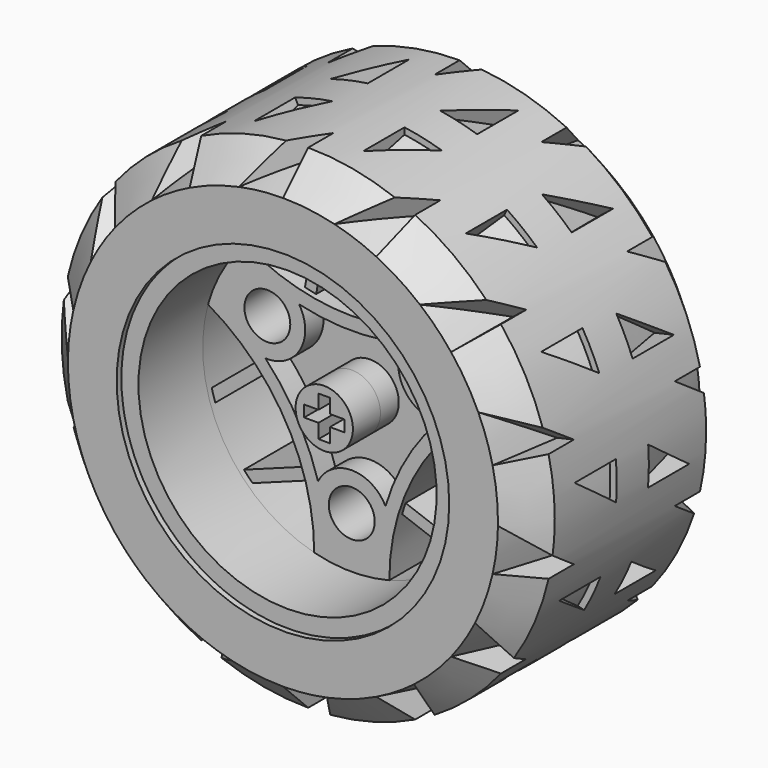
from build123d import *

# Parameters (mm, degrees)
F0_R             = 21.5
F0_R_2           = 14.5
F1_DEPTH         = 11
F1_DEPTH_BACK    = 11
F6_DEPTH         = 3.5
F6_COPIES_COUNT  = 14
F9_COPIES_COUNT  = 2
F11_COPIES_COUNT = 2
F14_R            = 2
F15_DEPTH        = 25
F16_R            = 2.5
F17_DEPTH        = 3
F19_DEPTH        = 17.501
F20_R            = 2.5
F21_DEPTH        = 2
F24_DEPTH        = 6
F24_COPIES_COUNT = 3


# Not quite as in the source:
# - a pattern or mirror of a feature is missing from the dataset's text; its kind, count and spacing are read off the source's solid


with BuildPart() as f1:
    # F0 (on Front) → F1 (new body, two sides)
    with BuildSketch(Plane.XZ) as f1_sk:
        Circle(F0_R)
        Circle(F0_R_2, mode=Mode.SUBTRACT)
    extrude(amount=F1_DEPTH)
    extrude(f1_sk.sketch, amount=-F1_DEPTH_BACK)

    # F3 (on offset) → F6 (cut)
    with BuildSketch(Plane.XY.offset(21.5)):
        Polygon((-3.8511414602, -11), (0, -11), (0, -5.5), align=None)
        Polygon((6.25, -1.5), (3, -1.5), (3, -6), align=None)
        Polygon((3.8511414602, 11), (0, 11), (0, 5.5), align=None)
        Polygon((-3, 2), (-3, 6.5), (-6.25, 2), align=None)
    f6 = extrude(amount=-F6_DEPTH, mode=Mode.SUBTRACT)

    # F6_copies: F6 ×14 about axis
    f6_copies_axis = Axis((0, 0, 0), (0, 1, 0))
    for i in range(1, F6_COPIES_COUNT):
        add(f6.rotate(f6_copies_axis, i * 360 / F6_COPIES_COUNT), mode=Mode.SUBTRACT)

    # F8 (on Right) → F9 (revolve, cut)
    with BuildSketch(Plane.YZ):
        Polygon((-11, 21.5), (-11, 18.75), (-8.25, 21.5), align=None)
    f9 = revolve(axis=Axis((0, -11, 0), (0, -1, 0)), mode=Mode.SUBTRACT)

    # F9_copies: F9 ×2 about axis
    f9_copies_axis = Axis((0, 0, 0), (0, 0, 1))
    for i in range(1, F9_COPIES_COUNT):
        add(f9.rotate(f9_copies_axis, i * 360 / F9_COPIES_COUNT), mode=Mode.SUBTRACT)

    # F10 (on Right) → F11 (revolve)
    with BuildSketch(Plane.YZ):
        Polygon((0, 21.289668856), (-11, 18.75), (-11, 18), (0, 18), align=None)
    f11 = revolve(axis=Axis((0, -11, 0), (0, -1, 0)))

    # F11_copies: F11 ×2 about axis
    f11_copies_axis = Axis((0, 0, 0), (0, 0, 1))
    for i in range(1, F11_COPIES_COUNT):
        add(f11.rotate(f11_copies_axis, i * 360 / F11_COPIES_COUNT))


with BuildPart() as f13:
    # F12 (on Right) → F13 (revolve)
    with BuildSketch(Plane.YZ):
        Polygon((10.5, 14.5), (-10.5, 14.5), (-10.5, 13), (-3.5, 13), (-3.5, 0), (3.5, 0), (3.5, 13), (10.5, 13), align=None)
    revolve(axis=Axis((0, 0, 0), (0, 1, 0)))

    # F14 (on face) → F15 (cut)
    with BuildSketch(Plane.XZ.offset(3.5)):
        with BuildLine():
            ThreePointArc((9.2577182745, 9.1265904011), (0, 13), (-9.2577182745, 9.1265904011))
            ThreePointArc((-9.2577182745, 9.1265904011), (-4.7921476073, 7.276890467), (0, 6.6459922657))
            ThreePointArc((0, 6.6459922657), (4.7921476073, 7.276890467), (9.2577182745, 9.1265904011))
        make_face()
        with BuildLine():
            ThreePointArc((-12.5327182745, 3.4541240063), (-11.2583302492, -6.5), (-3.275, -12.5807144074))
            ThreePointArc((-3.275, -12.5807144074), (-5.7555981354, -3.3229961328), (-12.5327182745, 3.4541240063))
        make_face()
        with BuildLine():
            ThreePointArc((3.275, -12.5807144074), (11.2583302492, -6.5), (12.5327182745, 3.4541240063))
            ThreePointArc((12.5327182745, 3.4541240063), (5.7555981354, -3.3229961328), (3.275, -12.5807144074))
        make_face()
        with Locations((7.3612159322, 4.25)):
            Circle(F14_R)
        with Locations((-7.3612159322, 4.25)):
            Circle(F14_R)
        with Locations((0, -8.5)):
            Circle(F14_R)
    extrude(amount=-F15_DEPTH, mode=Mode.SUBTRACT)

    # F16 (on face) → F17 (join)
    with BuildSketch(Plane.XZ.offset(3.5)):
        Circle(F16_R)
    f17 = extrude(amount=F17_DEPTH)

    # F17_copies: F17 across plane
    add(f17.mirror(Plane.ZX))

    # F18 (on face) → F19 (cut, through all)
    with BuildSketch(Plane.XZ.offset(6.5)):
        Polygon((-0.5, 1.75), (-0.5, 0.5), (-1.75, 0.5), (-1.75, -0.5), (-0.5, -0.5), (-0.5, -1.75), (0.5, -1.75), (0.5, -0.5), (1.75, -0.5), (1.75, 0.5), (0.5, 0.5), (0.5, 1.75), align=None)
    extrude(amount=-F19_DEPTH, mode=Mode.SUBTRACT)

    # F20 (on face) → F21 (cut)
    with BuildSketch(Plane(origin=(0, 3.5, 0), x_dir=(-1, 0, 0), z_dir=(0, 1, 0))):
        with BuildLine():
            ThreePointArc((-4.5907207549, 6.0486384092), (-4.5006114959, 2.5984292587), (-7.5336348981, 0.9513615908))
            ThreePointArc((-7.5336348981, 0.9513615908), (-4.7675077293, -2.7525218709), (-2.9429141432, -7))
            ThreePointArc((-2.9429141432, -7), (0, -5.1968585174), (2.9429141432, -7))
            ThreePointArc((2.9429141432, -7), (4.7675077293, -2.7525218709), (7.5336348981, 0.9513615908))
            ThreePointArc((7.5336348981, 0.9513615908), (4.5006114959, 2.5984292587), (4.5907207549, 6.0486384092))
            ThreePointArc((4.5907207549, 6.0486384092), (0, 5.5050437418), (-4.5907207549, 6.0486384092))
        make_face()
        Circle(F20_R, mode=Mode.SUBTRACT)
    f21 = extrude(amount=-F21_DEPTH, mode=Mode.SUBTRACT)

    # F21_copies: F21 across plane
    add(f21.mirror(Plane(origin=(0, 0, 0), x_dir=(0, 0, -1), z_dir=(0, -1, 0))), mode=Mode.SUBTRACT)

    # F23 (on offset) → F24 (join)
    with BuildSketch(Plane.XZ.offset(3)):
        with BuildLine():
            Line((-3.558824997, 12.5033901259), (-4.4775283372, 7.1955408436))
            ThreePointArc((-4.4775283372, 7.1955408436), (-3.990222415, 7.0810661059), (-3.5, 6.9798064833))
            Line((-3.5, 6.9798064833), (-2.5, 12.7573508222))
            ThreePointArc((-2.5, 12.7573508222), (-3.0320725741, 12.6414609878), (-3.558824997, 12.5033901259))
        make_face()
        with BuildLine():
            Line((2.5, 12.7573508222), (3.5, 6.9798064833))
            ThreePointArc((3.5, 6.9798064833), (3.990222415, 7.0810661059), (4.4775283372, 7.1955408436))
            Line((4.4775283372, 7.1955408436), (3.558824997, 12.5033901259))
            ThreePointArc((3.558824997, 12.5033901259), (3.0320725741, 12.6414609878), (2.5, 12.7573508222))
        make_face()
    f24 = extrude(amount=-F24_DEPTH)

    # F24_copies: F24 ×3 about axis
    f24_copies_axis = Axis((0, 0, 0), (0, 1, 0))
    for i in range(1, F24_COPIES_COUNT):
        add(f24.rotate(f24_copies_axis, i * 360 / F24_COPIES_COUNT))


solid = Compound([f1.part, f13.part])
